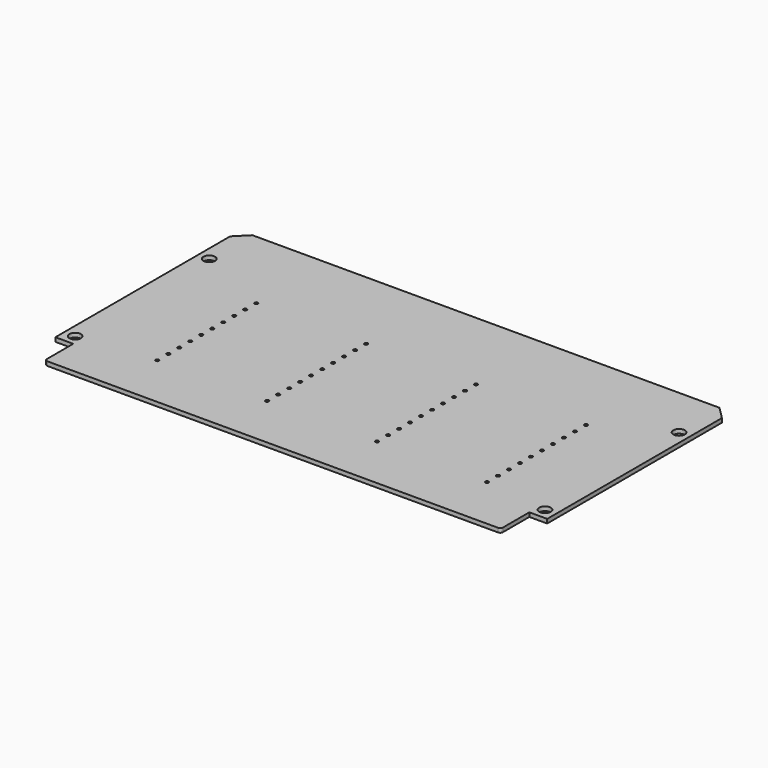
from build123d import *

# Parameters (mm, degrees)
F1_DEPTH = 1.5
F2_R     = 2.1
F2_R_2   = 0.6
F3_DEPTH = 1.501


# Not quite as in the source:
# - a feature names something its author has since deleted; it is built from what else it names


with BuildPart() as f1:
    # F0 (on Top) → F1 (new body)
    with BuildSketch(Plane.XY):
        with BuildLine():
            Line((83, -42), (-83, -42))
            Line((-83, -42), (-83, -54))
            ThreePointArc((-83, -54), (-82.7071067812, -54.7071067812), (-82, -55))
            Line((-82, -55), (82, -55))
            ThreePointArc((82, -55), (82.7071067812, -54.7071067812), (83, -54))
            Line((83, -54), (83, -42))
        make_face()
        Polygon((89.5, 42), (-89.5, 42), (-89.5, -42), (-83, -42), (83, -42), (89.5, -42), align=None)
    extrude(amount=F1_DEPTH)

    # F2 (on face) → F3 (cut, through all)
    with BuildSketch(Plane.XY.offset(1.5)):
        with Locations((-85.5, -38)):
            Circle(F2_R)
        with Locations((-85.5, 23)):
            Circle(F2_R)
        Polygon((-89.5, 42), (-89.5, 37.5), (-85, 42), align=None)
        with Locations((85.5, -38)):
            Circle(F2_R)
        Polygon((89.5, 42), (85, 42), (89.5, 37.5), align=None)
        with Locations((85.5, 23)):
            Circle(F2_R)
        with Locations((-58, -35)):
            Circle(F2_R_2)
        with Locations((-58, -30)):
            Circle(F2_R_2)
        with Locations((-58, -25)):
            Circle(F2_R_2)
        with Locations((-58, -20)):
            Circle(F2_R_2)
        with Locations((-58, -15)):
            Circle(F2_R_2)
        with Locations((-58, -10)):
            Circle(F2_R_2)
        with Locations((-58, -5)):
            Circle(F2_R_2)
        with Locations((-58, 0)):
            Circle(F2_R_2)
        with Locations((-58, 5)):
            Circle(F2_R_2)
        with Locations((-58, 10)):
            Circle(F2_R_2)
        with Locations((-18, 10)):
            Circle(F2_R_2)
        with Locations((-18, 5)):
            Circle(F2_R_2)
        with Locations((-18, 0)):
            Circle(F2_R_2)
        with Locations((-18, -5)):
            Circle(F2_R_2)
        with Locations((-18, -10)):
            Circle(F2_R_2)
        with Locations((-18, -15)):
            Circle(F2_R_2)
        with Locations((-18, -20)):
            Circle(F2_R_2)
        with Locations((-18, -25)):
            Circle(F2_R_2)
        with Locations((-18, -30)):
            Circle(F2_R_2)
        with Locations((-18, -35)):
            Circle(F2_R_2)
        with Locations((22, -35)):
            Circle(F2_R_2)
        with Locations((22, -30)):
            Circle(F2_R_2)
        with Locations((22, -25)):
            Circle(F2_R_2)
        with Locations((22, -20)):
            Circle(F2_R_2)
        with Locations((22, -15)):
            Circle(F2_R_2)
        with Locations((22, -10)):
            Circle(F2_R_2)
        with Locations((22, -5)):
            Circle(F2_R_2)
        with Locations((22, 0)):
            Circle(F2_R_2)
        with Locations((22, 5)):
            Circle(F2_R_2)
        with Locations((22, 10)):
            Circle(F2_R_2)
        with Locations((62, 10)):
            Circle(F2_R_2)
        with Locations((62, 5)):
            Circle(F2_R_2)
        with Locations((62, 0)):
            Circle(F2_R_2)
        with Locations((62, -5)):
            Circle(F2_R_2)
        with Locations((62, -10)):
            Circle(F2_R_2)
        with Locations((62, -15)):
            Circle(F2_R_2)
        with Locations((62, -20)):
            Circle(F2_R_2)
        with Locations((62, -25)):
            Circle(F2_R_2)
        with Locations((62, -30)):
            Circle(F2_R_2)
        with Locations((62, -35)):
            Circle(F2_R_2)
    extrude(amount=-F3_DEPTH, mode=Mode.SUBTRACT)


solid = f1.part
